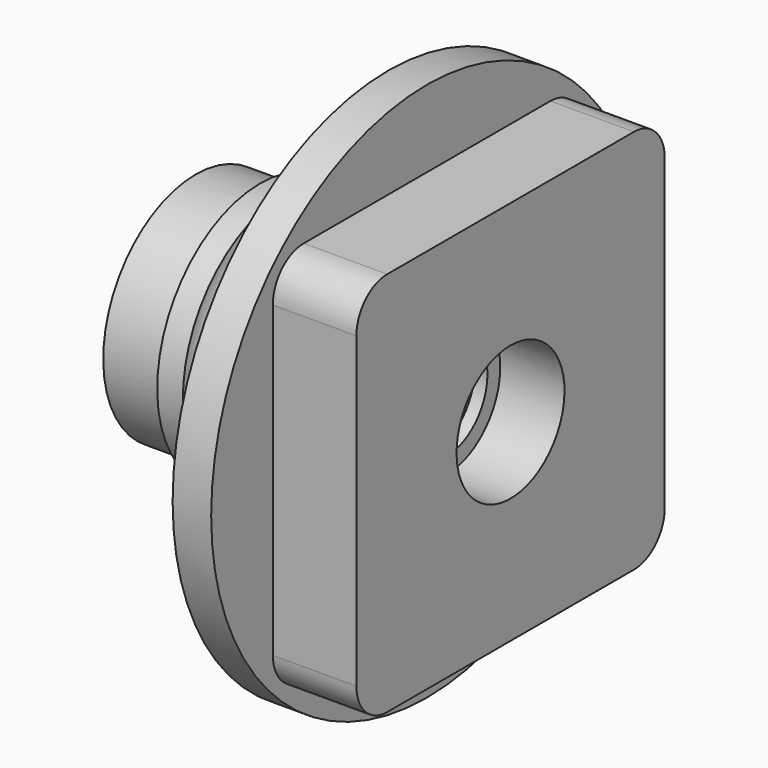
from build123d import *

# Parameters (mm, degrees)
F3_R        = 44
F3_W        = 60
F3_H        = 60
F4_DEPTH    = 13
F5_T1_DEPTH = 28


# Not quite as in the source:
# - a fillet or chamfer that OpenCascade refuses, or shapes differently, is made with other operations: its cross-section is extruded or revolved along the edge and cut away or added


with BuildPart() as f2:
    # F1 (on Front) → F2 (revolve)
    with BuildSketch(Plane.XZ):
        with BuildLine():
            Line((-18, 6), (0, 6))
            Line((0, 6), (7, 6))
            Line((7, 6), (7, 8))
            Line((7, 8), (9, 8))
            Line((9, 8), (9, 10.5))
            Line((9, 10.5), (19, 10.5))
            Line((19, 10.5), (19, 44))
            Line((19, 44), (6, 44))
            Line((6, 44), (6, 42))
            Line((6, 42), (0, 42))
            Line((0, 42), (0, 20))
            Line((0, 20), (-4, 20))
            ThreePointArc((-4, 20), (-10, 14), (-16, 20))
            Line((-16, 20), (-20, 20))
            Line((-20, 20), (-20, 18))
            Line((-20, 18), (-30, 18))
            Line((-30, 18), (-30, 10.5))
            Line((-30, 10.5), (-20, 10.5))
            Line((-20, 10.5), (-20, 8))
            Line((-20, 8), (-18, 8))
            Line((-18, 8), (-18, 6))
        make_face()
    revolve(axis=Axis((43.6499677598, 0, 0), (1, 0, 0)))

    # F3 (on face) → F4 (cut, through all)
    with BuildSketch(Plane.YZ.offset(19)):
        Circle(F3_R)
        Rectangle(F3_W, F3_H, mode=Mode.SUBTRACT)
    extrude(amount=-F4_DEPTH, mode=Mode.SUBTRACT)

    # F5: fillet of radius 6 on 4 edges, made by hand

    # F5_s2 → F5_t1 (cut)
    with BuildSketch(Plane.YZ.offset(6)):
        with BuildLine():
            ThreePointArc((-30, -24), (-28.2426406871, -28.2426406871), (-24, -30))
            Line((-24, -30), (-30, -30))
            Line((-30, -30), (-30, -24))
        make_face()
        with BuildLine():
            ThreePointArc((24, -30), (28.2426406871, -28.2426406871), (30, -24))
            Line((30, -24), (30, -30))
            Line((30, -30), (24, -30))
        make_face()
        with BuildLine():
            ThreePointArc((-30, 24), (-28.2426406871, 28.2426406871), (-24, 30))
            Line((-24, 30), (-30, 30))
            Line((-30, 30), (-30, 24))
        make_face()
        with BuildLine():
            ThreePointArc((30, 24), (28.2426406871, 28.2426406871), (24, 30))
            Line((24, 30), (30, 30))
            Line((30, 30), (30, 24))
        make_face()
    extrude(amount=F5_T1_DEPTH, mode=Mode.SUBTRACT)


solid = f2.part
